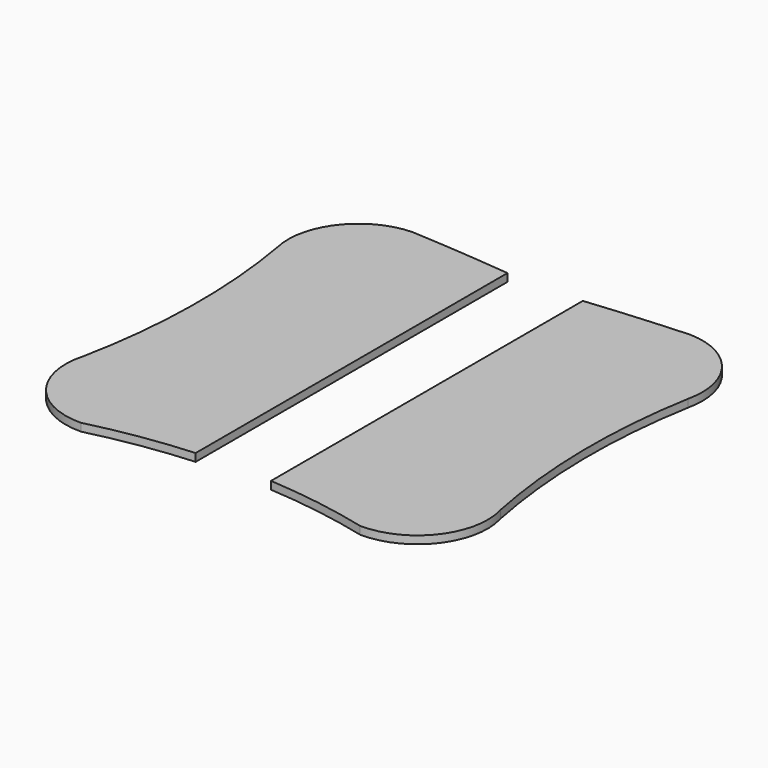
from build123d import *

# Parameters (mm, degrees)
F1_DEPTH = 25.4


# Not quite as in the source:
# - a feature names something its author has since deleted; it is built from what else it names


with BuildPart() as f1:
    # F0 (on Top) → F1 (new body)
    with BuildSketch(Plane.XY):
        with BuildLine():
            Line((-122.74547472, 363.4131123645), (-122.74547472, 617.4131123645))
            ThreePointArc((-122.74547472, 617.4131123645), (-287.6923004816, 632.1043774637), (-452.94547472, 642.8131123645))
            ThreePointArc((-452.94547472, 642.8131123645), (-626.8733109875, 554.0959858439), (-668.84547472, 363.4131123645))
            ThreePointArc((-668.84547472, 363.4131123645), (-637.6124772586, -25.6986468555), (-678.8013792429, -413.8827985761))
            ThreePointArc((-678.8013792429, -413.8827985761), (-639.8991633536, -615.573241104), (-454.793114458, -704.61349981))
            ThreePointArc((-454.793114458, -704.61349981), (-289.9406925994, -671.1240208892), (-122.74547472, -652.5868876355))
            Line((-122.74547472, -652.5868876355), (-122.74547472, 363.4131123645))
        make_face()
    extrude(amount=F1_DEPTH)


with BuildPart() as f2_1:
    # F2: instance of F1
    add(f1.part.mirror(Plane.YZ))


solid = Compound([f1.part, f2_1.part])
